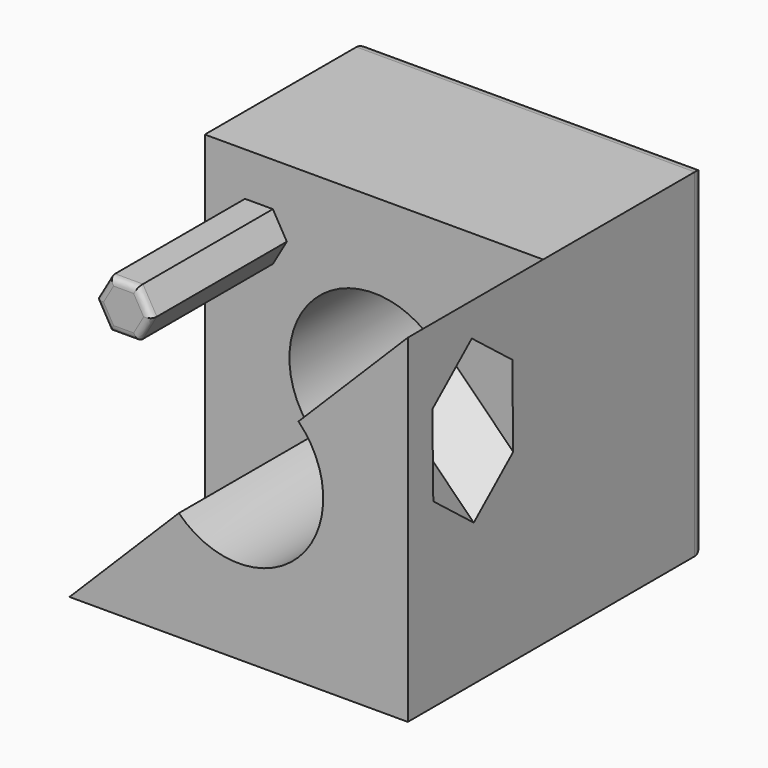
from build123d import *
from build123d import SkipClean  # not in build123d's __all__

# Parameters (mm, degrees)
F0_W        = 50
F0_H        = 50
F0_R        = 12.5
F1_DEPTH    = 30
F2_DEPTH    = 25
F4_DEPTH    = 25
F6_DEPTH    = 50
F8_DEPTH    = 25
F9_T1_DEPTH = 9.1191559928
F9_T3_DEPTH = 9.1191559928
F9_T5_DEPTH = 9.1191559928
F9_T7_DEPTH = 9.1191559928
F9_T9_DEPTH = 9.1191559928
F10_R       = 2


# Not quite as in the source:
# - a fillet or chamfer that OpenCascade refuses, or shapes differently, is made with other operations: its cross-section is extruded or revolved along the edge and cut away or added
# - after a boolean that leaves OpenCascade's solid faulty, fix() repairs it


with BuildPart() as f1:
    # F0 (on Front) → F1 (new body)
    with BuildSketch(Plane.XZ):
        Rectangle(F0_W, F0_H)
        Circle(F0_R, mode=Mode.SUBTRACT)
    extrude(amount=F1_DEPTH)

    # F0 (on Front) → F2 (join)
    with BuildSketch(Plane.XZ):
        Rectangle(F0_W, F0_H)
        Circle(F0_R, mode=Mode.SUBTRACT)
    extrude(amount=F2_DEPTH)

    # F3 (on face) → F4 (join)
    with BuildSketch(Plane.XZ.offset(30)):
        with BuildLine():
            Line((-8.8388347648, -8.8388347648), (-25, -25))
            Line((-25, -25), (25, -25))
            Line((25, -25), (25, 25))
            Line((25, 25), (8.8388347648, 8.8388347648))
            ThreePointArc((8.8388347648, 8.8388347648), (8.8388347648, -8.8388347648), (-8.8388347648, -8.8388347648))
        make_face()
    with SkipClean():  # cleaning this boolean's faces spoils the solid; the shape is the same uncleaned
        extrude(amount=F4_DEPTH)

    # F5 (on face) → F6 (cut)
    with BuildSketch(Plane(origin=(0, 0, 0), x_dir=(0.7071067812, 0, 0.7071067812), z_dir=(-0.7071067812, 0, 0.7071067812))):
        Polygon((-23.9276695297, -31), (-34.3199743751, -49), (-13.5353646843, -49), align=None)
        Polygon((19.249809042, -35.5263909924), (14.8302387921, -42.8186887872), (18.9357688095, -50.2922977948), (27.4608690767, -50.4736090076), (31.8804393265, -43.1813112128), (27.7749093092, -35.7077022052), align=None)
    extrude(amount=-F6_DEPTH, mode=Mode.SUBTRACT)

    add(f1.part.fix(), mode=Mode.REPLACE)

    # F7 (on face) → F8 (join)
    with BuildSketch(Plane.XZ.offset(30)):
        Polygon((-19.0595779964, 11.4327062681), (-14.9404220036, 11.4327062681), (-12.8808440072, 15), (-14.9404220036, 18.5672937319), (-19.0595779964, 18.5672937319), (-21.1191559928, 15), align=None)
    extrude(amount=F8_DEPTH)

    # F9: fillet of radius 1 on 6 edges, made by hand

    # F9_s2 → F9_t1 (cut)
    with BuildSketch(Plane(origin=(4.5249795266, 0, 7.8374944433), x_dir=(0, 1, 0), z_dir=(-0.5, 0, -0.8660254038))):
        with BuildLine():
            add(Edge.make_bspline(
                [(-54, -25.7897255963), (-55, -25.7897255963), (-55, -24.7897255963)],
                knots=[0, 0, 0, 1, 1, 1], degree=2, weights=[1, 1, 1]))
            Line((-55, -24.7897255963), (-55, -25.7897255963))
            Line((-55, -25.7897255963), (-54, -25.7897255963))
        make_face()
    extrude(amount=F9_T1_DEPTH, mode=Mode.SUBTRACT)

    # F9_s4 → F9_t3 (cut)
    with BuildSketch(Plane(origin=(-13.0249795266, 0, 22.5599263076), x_dir=(0, 1, 0), z_dir=(0.5, 0, -0.8660254038))):
        with BuildLine():
            add(Edge.make_bspline(
                [(-54, -10.7897255963), (-55, -10.7897255963), (-55, -9.7897255963)],
                knots=[0, 0, 0, 1, 1, 1], degree=2, weights=[1, 1, 1]))
            Line((-55, -9.7897255963), (-55, -10.7897255963))
            Line((-55, -10.7897255963), (-54, -10.7897255963))
        make_face()
    extrude(amount=F9_T3_DEPTH, mode=Mode.SUBTRACT)

    # F9_s6 → F9_t5 (cut)
    with BuildSketch(Plane.YZ.offset(-21.5595779964)):
        with BuildLine():
            add(Edge.make_bspline(
                [(-54, 11.4327062681), (-55, 11.4327062681), (-55, 12.4327062681)],
                knots=[0, 0, 0, 1, 1, 1], degree=2, weights=[1, 1, 1]))
            Line((-55, 12.4327062681), (-55, 11.4327062681))
            Line((-55, 11.4327062681), (-54, 11.4327062681))
        make_face()
        with BuildLine():
            add(Edge.make_bspline(
                [(-54, 18.5672937319), (-55, 18.5672937319), (-55, 17.5672937319)],
                knots=[0, 0, 0, 1, 1, 1], degree=2, weights=[1, 1, 1]))
            Line((-55, 17.5672937319), (-55, 18.5672937319))
            Line((-55, 18.5672937319), (-54, 18.5672937319))
        make_face()
    extrude(amount=F9_T5_DEPTH, mode=Mode.SUBTRACT)

    # F9_s8 → F9_t7 (cut)
    with BuildSketch(Plane(origin=(-0.0345984698, 0, -0.0599263076), x_dir=(0, 1, 0), z_dir=(0.5, 0, 0.8660254038))):
        with BuildLine():
            add(Edge.make_bspline(
                [(-54, 18.6551381324), (-55, 18.6551381324), (-55, 19.6551381324)],
                knots=[0, 0, 0, 1, 1, 1], degree=2, weights=[1, 1, 1]))
            Line((-55, 19.6551381324), (-55, 18.6551381324))
            Line((-55, 18.6551381324), (-54, 18.6551381324))
        make_face()
    extrude(amount=F9_T7_DEPTH, mode=Mode.SUBTRACT)

    # F9_s10 → F9_t9 (cut)
    with BuildSketch(Plane(origin=(-8.4654015302, 0, 14.6625055567), x_dir=(0, 1, 0), z_dir=(-0.5, 0, 0.8660254038))):
        with BuildLine():
            add(Edge.make_bspline(
                [(-54, 3.6551381324), (-55, 3.6551381324), (-55, 4.6551381324)],
                knots=[0, 0, 0, 1, 1, 1], degree=2, weights=[1, 1, 1]))
            Line((-55, 4.6551381324), (-55, 3.6551381324))
            Line((-55, 3.6551381324), (-54, 3.6551381324))
        make_face()
    extrude(amount=F9_T9_DEPTH, mode=Mode.SUBTRACT)

    # F10
    f10_edges = [f1.edges().sort_by_distance(p)[0] for p in [
        (25, 0, 0),
        (0, 0, -25),
        (-25, 0, 0),
        (0, 0, 25),
    ]]
    fillet(f10_edges, radius=F10_R)


solid = f1.part
